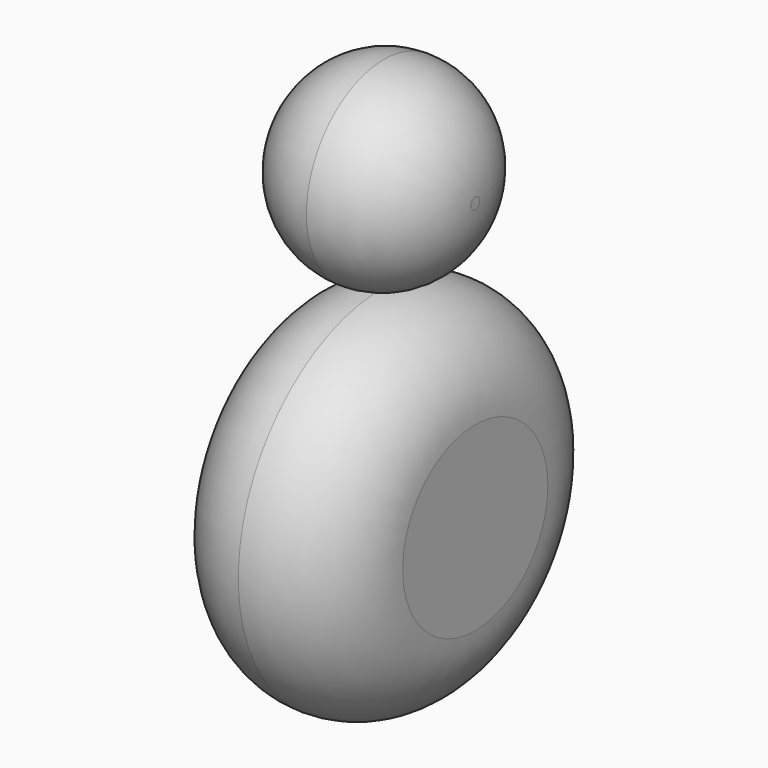
from build123d import *

# Parameters (mm, degrees)
F0_R     = 25.3209330863
F1_DEPTH = 25.4
F2_R     = 12.69999
F3_R     = 13.4789007608
F4_DEPTH = 25.4
F5_R     = 12.69999


# Not quite as in the source:
# - a fillet or chamfer is up to 0.001 mm smaller than in the source, because OpenCascade refuses the exact size


with BuildPart() as f1:
    # F0 (on Right) → F1 (new body)
    with BuildSketch(Plane.YZ):
        Circle(F0_R)
    extrude(amount=F1_DEPTH)

    # F2 (radius 12.7 in the source; OpenCascade refuses exactly that, so slightly less here)
    f2_edges = [f1.edges().sort_by_distance(p)[0] for p in [
        (12.7, 25.320933, 0),
        (0, -25.320933, 0),
        (25.4, -25.320933, 0),
    ]]
    fillet(f2_edges, radius=F2_R)


with BuildPart() as f4:
    # F3 (on Right) → F4 (new body)
    with BuildSketch(Plane.YZ):
        with Locations((0, 39.7534705698)):
            Circle(F3_R)
    extrude(amount=F4_DEPTH)

    # F5 (radius 12.7 in the source; OpenCascade refuses exactly that, so slightly less here)
    f5_edges = [f4.edges().sort_by_distance(p)[0] for p in [
        (12.7, 13.478901, 39.753471),
        (0, -13.478901, 39.753471),
        (25.4, -13.478901, 39.753471),
    ]]
    fillet(f5_edges, radius=F5_R)


solid = Compound([f1.part, f4.part])
